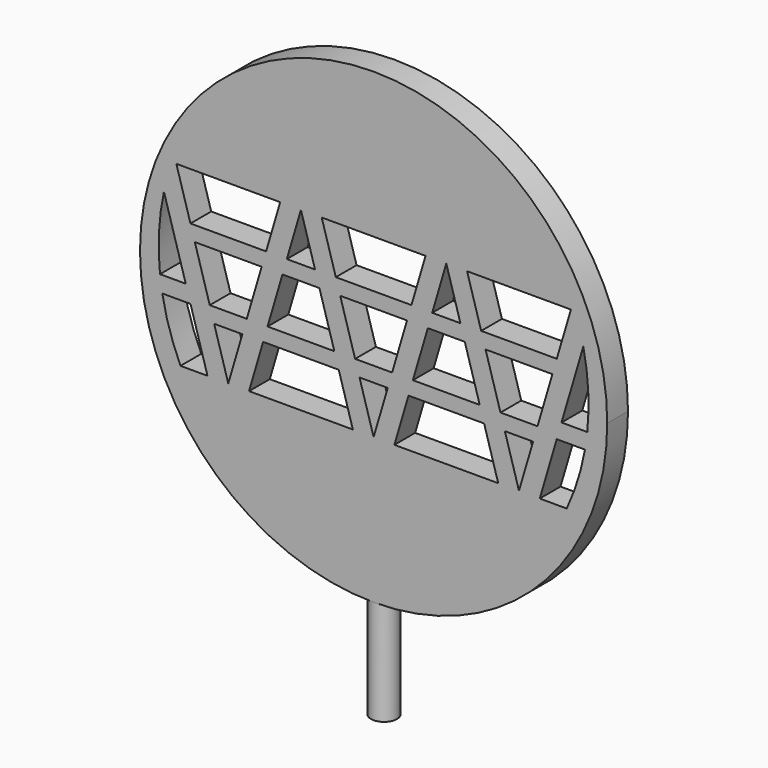
from build123d import *
from build123d import SkipClean  # not in build123d's __all__

# Parameters (mm, degrees)
F0_R     = 45
F1_DEPTH = 5
F2_R     = 2.5
F3_DEPTH = 65
F7_DEPTH = 5.0010001144


# Not quite as in the source:
# - a feature of the source that left no trace in its solid (it failed there, or was rolled back) is left out
# - a feature names something its author has since deleted; it is built from what else it names


with BuildPart() as f1:
    # F0 (on Front) → F1 (new body)
    with BuildSketch(Plane.XZ):
        Circle(F0_R)
    extrude(amount=F1_DEPTH)

    # F2 (on Top) → F3 (join)
    with BuildSketch(Plane.XY):
        with Locations((0, -2.5)):
            Circle(F2_R)
    with SkipClean():  # cleaning this boolean's faces spoils the solid; the shape is the same uncleaned
        extrude(amount=-F3_DEPTH)

    # F6 (on face) → F7 (cut, through all)
    with BuildSketch(Plane.XZ.offset(5)):
        Polygon((-20.7163122443, 7.7645383693), (-18, 17), (-38, 17), (-35.2836877557, 7.7645383693), align=None)
        with BuildLine():
            Line((-36.1941438848, -2.7399107917), (-40.3882877696, 11.5201784167))
            ThreePointArc((-40.3882877696, 11.5201784167), (-41.3363102402, 4.4204212554), (-41.1493788917, -2.7399107917))
            Line((-41.1493788917, -2.7399107917), (-36.1941438848, -2.7399107917))
        make_face()
        with BuildLine():
            Line((-32, -17), (-35.2739794285, -5.8684699433))
            Line((-35.2739794285, -5.8684699433), (-40.7068101942, -5.8684699433))
            ThreePointArc((-40.7068101942, -5.8684699433), (-39.3148104816, -11.548035888), (-37.2002845672, -17))
            Line((-37.2002845672, -17), (-32, -17))
        make_face()
        Polygon((-24.4349641852, -4.8788782297), (-21.5628112163, 4.8864418646), (-34.4371887837, 4.8864418646), (-31.5650358148, -4.8788782297), align=None)
        Polygon((-28, -17), (-25.2814631572, -7.7569747344), (-30.7185368428, -7.7569747344), align=None)
        Polygon((-11.2836877557, 7.7645383693), (-14, 17), (-16.7163122443, 7.7645383693), align=None)
        Polygon((-7.5650358148, -4.8788782297), (-10.4371887837, 4.8864418646), (-17.5628112163, 4.8864418646), (-20.4349641852, -4.8788782297), align=None)
        Polygon((-4, -17), (-6.7185368428, -7.7569747344), (-21.2814631572, -7.7569747344), (-24, -17), align=None)
        Polygon((0, -7.7569747344), (-2.7185368428, -7.7569747344), (0, -17), align=None)
        Polygon((0, -7.7569747344), (0, -17), (2.7185368428, -7.7569747344), align=None)
        Polygon((6.4371887837, 4.8864418646), (0, 4.8864418646), (0, 0), (0, -4.8788782297), (3.5650358148, -4.8788782297), align=None)
        Polygon((0, 4.8864418646), (-6.4371887837, 4.8864418646), (-3.5650358148, -4.8788782297), (0, -4.8788782297), (0, 0), align=None)
        Polygon((0, 17), (-10, 17), (-7.2836877557, 7.7645383693), (0, 7.7645383693), align=None)
        Polygon((10, 17), (0, 17), (0, 7.7645383693), (7.2836877557, 7.7645383693), align=None)
        Polygon((16.7163122443, 7.7645383693), (14, 17), (11.2836877557, 7.7645383693), align=None)
        Polygon((17.5628112163, 4.8864418646), (10.4371887837, 4.8864418646), (7.5650358148, -4.8788782297), (20.4349641852, -4.8788782297), align=None)
        Polygon((21.2814631572, -7.7569747344), (6.7185368428, -7.7569747344), (4, -17), (24, -17), align=None)
        Polygon((25.2814631572, -7.7569747344), (28, -17), (30.7185368428, -7.7569747344), align=None)
        Polygon((24.4349641852, -4.8788782297), (31.5650358148, -4.8788782297), (34.4371887837, 4.8864418646), (21.5628112163, 4.8864418646), align=None)
        Polygon((20.7163122443, 7.7645383693), (35.2836877557, 7.7645383693), (38, 17), (18, 17), align=None)
        with BuildLine():
            ThreePointArc((41.1493788917, -2.7399107917), (41.3363102402, 4.4204212554), (40.3882877696, 11.5201784167))
            Line((40.3882877696, 11.5201784167), (36.1941438848, -2.7399107917))
            Line((36.1941438848, -2.7399107917), (41.1493788917, -2.7399107917))
        make_face()
        with BuildLine():
            Line((40.7068101942, -5.8684699433), (35.2739794285, -5.8684699433))
            Line((35.2739794285, -5.8684699433), (32, -17))
            Line((32, -17), (37.2002845672, -17))
            ThreePointArc((37.2002845672, -17), (39.3148104816, -11.548035888), (40.7068101942, -5.8684699433))
        make_face()
    with SkipClean():  # cleaning this boolean's faces spoils the solid; the shape is the same uncleaned
        extrude(amount=-F7_DEPTH, mode=Mode.SUBTRACT)


solid = f1.part
